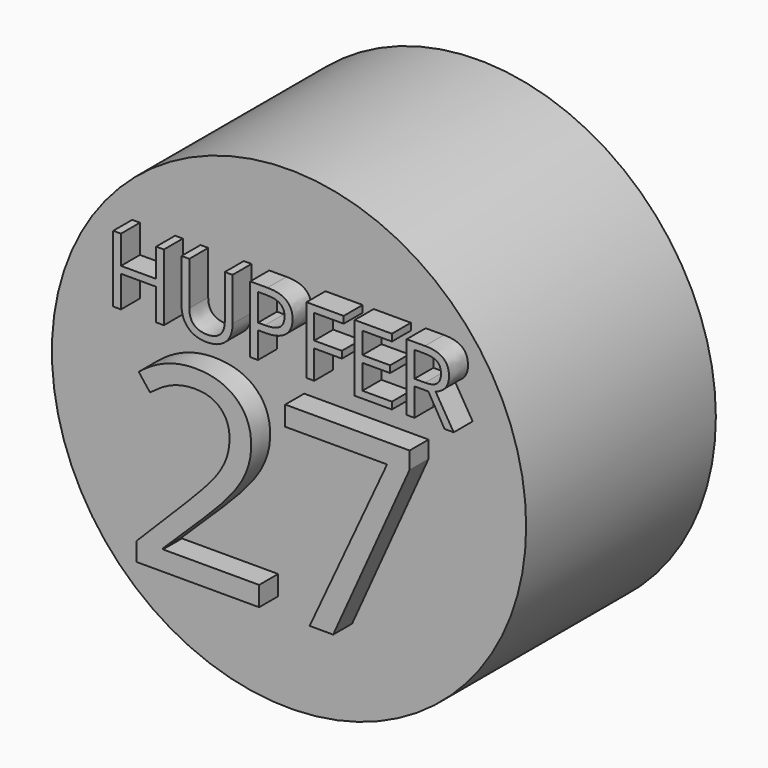
from build123d import *

# Parameters (mm, degrees)
F0_R         = 12.7
F1_DEPTH     = 12.7
F2_TEXT_SIZE = 5.0053370556
F3_DEPTH     = 1.27
F4_TEXT_SIZE = 14.0222081271
F5_DEPTH     = 1.27


# Not quite as in the source:
# - Text() gives the source's letters only with a copy of the font that has no kerning and outlines rounded to 1/6400 em; it was checked with that copy


with BuildPart() as f1:
    # F0 (on Front) → F1 (new body)
    with BuildSketch(Plane.XZ):
        with Locations((-15.1898693293, 33.2372374833)):
            Circle(F0_R)
    extrude(amount=F1_DEPTH)

    # F2 (on face) → F3 (join)
    with BuildSketch(Plane.XZ.offset(12.7)):
        with Locations((-24.0798693293, 37.2533948032)):
            Text('HUPFER', F2_TEXT_SIZE, font='Open Sans', text_align=(TextAlign.LEFT, TextAlign.BOTTOM))
    extrude(amount=F3_DEPTH)

    # F4 (on face) → F5 (join)
    with BuildSketch(Plane.XZ.offset(12.7)):
        with Locations((-23.0385752364, 25.6172374833)):
            Text('27', F4_TEXT_SIZE, font='Open Sans', text_align=(TextAlign.LEFT, TextAlign.BOTTOM))
    extrude(amount=F5_DEPTH)


solid = f1.part
